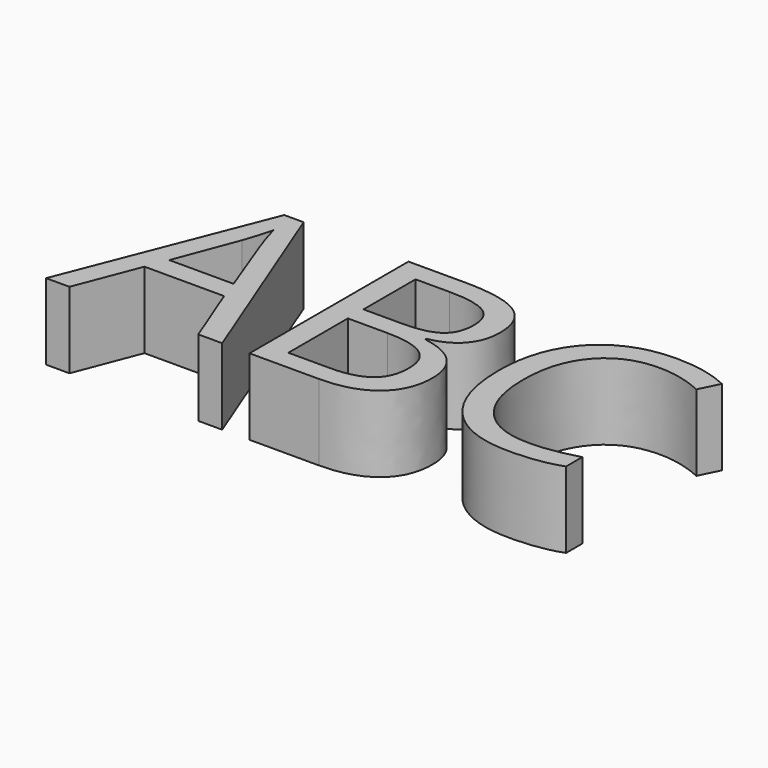
from build123d import *

# Parameters (mm, degrees)
F0_TEXT_SIZE = 92.8139546886
F1_DEPTH     = 25.4


# Not quite as in the source:
# - Text() gives the source's letters only with a copy of the font that has no kerning and outlines rounded to 1/6400 em; it was checked with that copy


with BuildPart() as f1:
    # F0 (on Top) → F1 (new body)
    with BuildSketch(Plane.XY):
        with Locations((-51.278963685, -79.5845687389)):
            Text('ABC', F0_TEXT_SIZE, font='Open Sans', text_align=(TextAlign.LEFT, TextAlign.BOTTOM))
    extrude(amount=F1_DEPTH)


solid = f1.part
